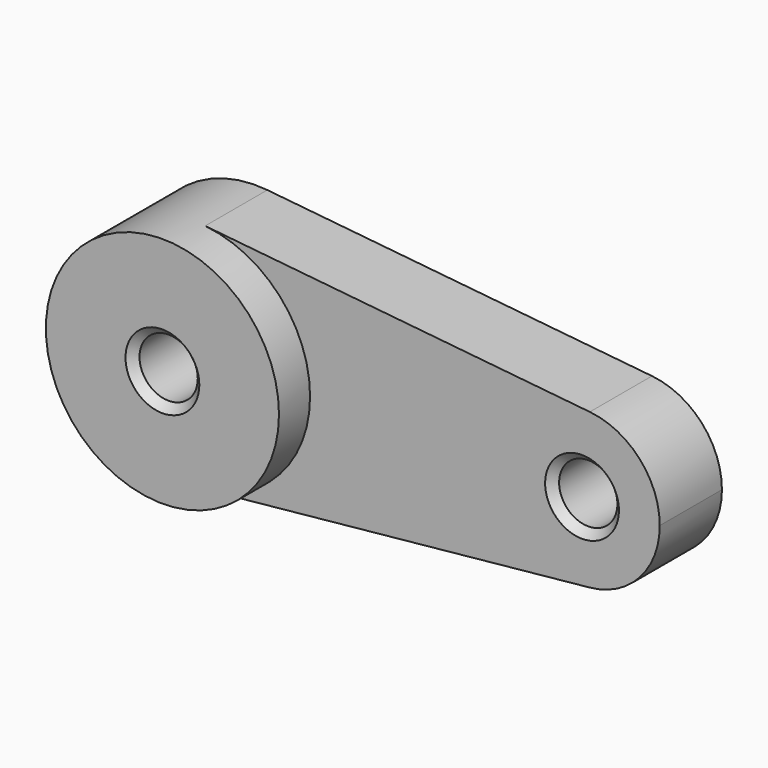
from build123d import *

# Parameters (mm, degrees)
F1_R     = 9.525
F2_DEPTH = 25.4
F0_R     = 38.1
F0_R_2   = 9.525
F3_DEPTH = 38.1
F4_SIZE  = 2.54


with BuildPart() as f2:
    # F1 (on face) → F2 (new body)
    with BuildSketch(Plane.XZ):
        with BuildLine():
            ThreePointArc((-13.4022655529, 0), (-23.2465491404, 25.5582567875), (-47.6922650288, 37.9090213011))
            ThreePointArc((-47.6922650288, 37.9090213011), (-89.6022655529, 2.206e-07), (-47.6922654678, -37.9090213452))
            ThreePointArc((-47.6922654678, -37.9090213452), (-23.2465492884, -25.5582569511), (-13.4022655529, 0))
        make_face()
        with Locations((-51.5022655529, 0)):
            Circle(F1_R, mode=Mode.SUBTRACT)
        with BuildLine():
            Line((78.0377345258, 25.2726808946), (-47.6922650288, 37.9090213011))
            ThreePointArc((-47.6922650288, 37.9090213011), (-23.2465491404, 25.5582567875), (-13.4022655529, 0))
            ThreePointArc((-13.4022655529, 0), (-23.2465492884, -25.5582569511), (-47.6922654678, -37.9090213452))
            Line((-47.6922654678, -37.9090213452), (78.0377338702, -25.2726809605))
            ThreePointArc((78.0377338702, -25.2726809605), (50.0977344471, 3.295e-07), (78.0377345258, 25.2726808946))
        make_face()
        with BuildLine():
            ThreePointArc((100.8977344471, 0), (94.3348786309, 17.0388379592), (78.0377345258, 25.2726808946))
            ThreePointArc((78.0377345258, 25.2726808946), (50.0977344471, 3.295e-07), (78.0377338702, -25.2726809605))
            ThreePointArc((78.0377338702, -25.2726809605), (94.3348784099, -17.0388382036), (100.8977344471, 0))
        make_face()
        with Locations((75.4977344471, 0)):
            Circle(F1_R, mode=Mode.SUBTRACT)
    extrude(amount=F2_DEPTH)

    # F0 (on Front) → F3 (join)
    with BuildSketch(Plane.XZ):
        with Locations((-51.5022655529, 0)):
            Circle(F0_R)
        with Locations((-51.5022655529, 0)):
            Circle(F0_R_2, mode=Mode.SUBTRACT)
    extrude(amount=F3_DEPTH)

    # F4
    f4_edges = [f2.edges().sort_by_distance(p)[0] for p in [
        (85.022734, -12.7, 0),
        (65.972734, 0, 0),
        (65.972734, -25.4, 0),
        (-61.027266, 0, 0),
        (-41.977266, -19.05, 0),
        (-61.027266, -38.1, 0),
    ]]
    chamfer(f4_edges, length=F4_SIZE)


solid = f2.part
